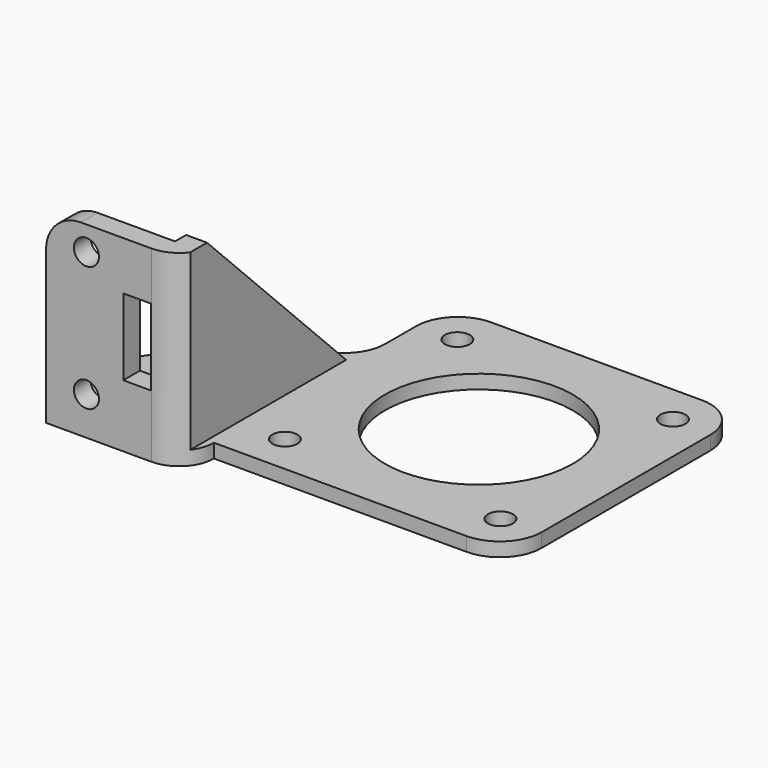
from build123d import *

# Parameters (mm, degrees)
F0_R         = 1.8
F0_R_2       = 13.5
F0_W         = 20.1372796029
F0_H         = 5
F1_DEPTH     = 2
F2_W         = 3
F2_H         = 30
F3_DEPTH     = 27
F4_W         = 16.1372796029
F4_H         = 3
F5_DEPTH     = 25
F6_R         = 1.8
F6_W         = 4
F6_H         = 11
F7_DEPTH     = 25
F8_SIZE      = 25
F9_SIZE      = 14
F10_R        = 4.99999
F11_T1_DEPTH = 2
F11_T3_DEPTH = 32


# Not quite as in the source:
# - a fillet or chamfer that OpenCascade refuses, or shapes differently, is made with other operations: its cross-section is extruded or revolved along the edge and cut away or added
# - a fillet or chamfer is up to 0.001 mm smaller than in the source, because OpenCascade refuses the exact size
# - a feature names something its author has since deleted; it is built from what else it names


with BuildPart() as f1:
    # F0 (on Top) → F1 (new body)
    with BuildSketch(Plane.XY):
        Polygon((21.15, -21.15), (21.15, 21.15), (-21.15, 21.15), (-21.15, 3.85), (-21.15, -21.15), align=None)
        with Locations((-15.5, -15.5)):
            Circle(F0_R, mode=Mode.SUBTRACT)
        with Locations((15.5, -15.5)):
            Circle(F0_R, mode=Mode.SUBTRACT)
        with Locations((-15.5, 15.5)):
            Circle(F0_R, mode=Mode.SUBTRACT)
        Circle(F0_R_2, mode=Mode.SUBTRACT)
        with Locations((15.5, 15.5)):
            Circle(F0_R, mode=Mode.SUBTRACT)
        Polygon((-21.15, -21.15), (-21.15, 3.85), (-41.3, 3.85), (-41.3, -21.15), (-21.1627203971, -21.15), align=None)
        with Locations((-31.2313601986, -23.65)):
            Rectangle(F0_W, F0_H)
    extrude(amount=F1_DEPTH)

    # F2 (on Top) → F3 (join)
    with BuildSketch(Plane.XY):
        with Locations((-23.6627203971, -11.15)):
            Rectangle(F2_W, F2_H)
    extrude(amount=F3_DEPTH)

    # F4 (on face) → F5 (join)
    with BuildSketch(Plane.XY.offset(2)):
        with Locations((-33.2313601986, -24.65)):
            Rectangle(F4_W, F4_H)
    extrude(amount=F5_DEPTH)

    # F6 (on face) → F7 (cut)
    with BuildSketch(Plane(origin=(0, -23.15, 0), x_dir=(-1, 0, 0), z_dir=(0, 1, 0))):
        with Locations((35.5, 5.5)):
            Circle(F6_R)
        with Locations((35.5, 23.5)):
            Circle(F6_R)
        with Locations((28.2, 14.5)):
            Rectangle(F6_W, F6_H)
    extrude(amount=-F7_DEPTH, mode=Mode.SUBTRACT)

    # F8
    f8_edges = [f1.edges().sort_by_distance(p)[0] for p in [
        (-23.66272, 3.85, 27),
    ]]
    chamfer(f8_edges, length=F8_SIZE)

    # F9
    f9_edges = [f1.edges().sort_by_distance(p)[0] for p in [
        (-41.3, 3.85, 1),
    ]]
    chamfer(f9_edges, length=F9_SIZE)

    # F10 (radius 5 in the source; OpenCascade refuses exactly that, so slightly less here)
    f10_edges = [f1.edges().sort_by_distance(p)[0] for p in [
        (-41.3, -10.15, 1),
        (-27.3, 3.85, 1),
        (-21.16272, -26.15, 1),
        (-41.3, -24.65, 27),
    ]]
    fillet(f10_edges, radius=F10_R)

    # F11: fillet of radius 6 on 4 edges, made by hand

    # F11_s2 → F11_t1 (join)
    with BuildSketch(Plane.XY):
        with BuildLine():
            ThreePointArc((-26.1021461366, 3.7731598692), (-22.5517871308, 5.8265464621), (-21.15, 9.6809515277))
            Line((-21.15, 9.6809515277), (-20.55, 9.6809515277))
            Line((-20.55, 9.6809515277), (-20.55, 3.85))
            Line((-20.55, 3.85), (-21.15, 3.25))
            ThreePointArc((-21.15, 3.25), (-25.2289363303, 3.25), (-25.9973607503, 3.1823807033))
            Line((-25.9973607503, 3.1823807033), (-26.1021461366, 3.7731598692))
        make_face()
    extrude(amount=F11_T1_DEPTH)

    # F11_s4 → F11_t3 (cut)
    with BuildSketch(Plane.XY.offset(-15)):
        with BuildLine():
            ThreePointArc((21.15, -15.15), (19.3926406871, -19.3926406871), (15.15, -21.15))
            Line((15.15, -21.15), (21.15, -21.15))
            Line((21.15, -21.15), (21.15, -15.15))
        make_face()
        with BuildLine():
            ThreePointArc((15.15, 21.15), (19.3926406871, 19.3926406871), (21.15, 15.15))
            Line((21.15, 15.15), (21.15, 21.15))
            Line((21.15, 21.15), (15.15, 21.15))
        make_face()
        with BuildLine():
            ThreePointArc((-21.15, 15.15), (-19.3926406871, 19.3926406871), (-15.15, 21.15))
            Line((-15.15, 21.15), (-21.15, 21.15))
            Line((-21.15, 21.15), (-21.15, 15.15))
        make_face()
    extrude(amount=F11_T3_DEPTH, mode=Mode.SUBTRACT)


solid = f1.part
